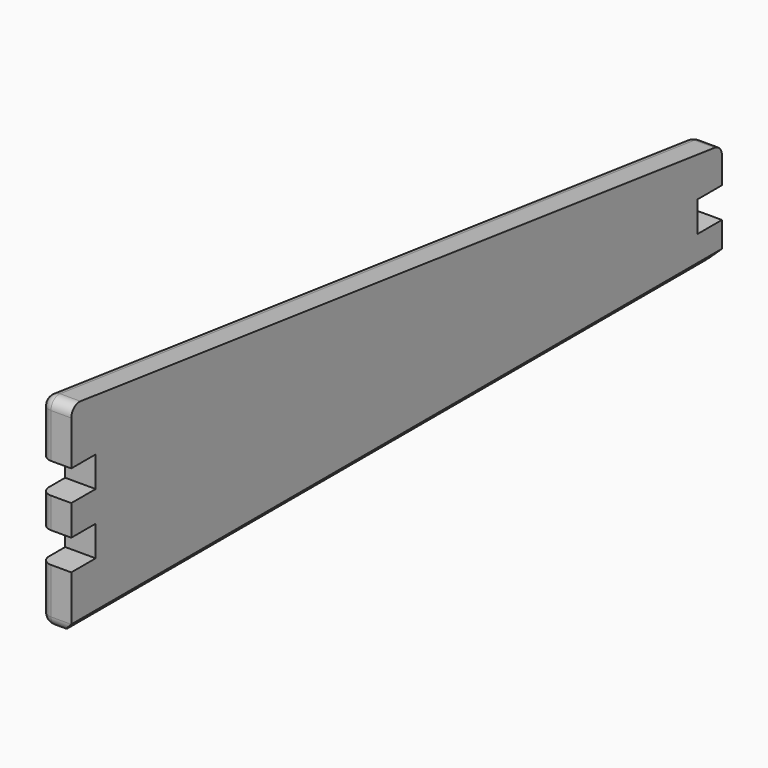
from build123d import *

# Parameters (mm, degrees)
F1_DEPTH     = 15
F2_R         = 5
F3_T1_DEPTH  = 390
F3_T3_DEPTH  = 393.0350652296
F3_T5_DEPTH  = 22.5
F3_T7_DEPTH  = 21.0347777317
F3_T9_DEPTH  = 24.1597777317
F3_T14_DEPTH = 5
F3_T20_DEPTH = 5
F3_T24_ANGLE = 90
F3_T26_ANGLE = 90
F4_T1_DEPTH  = 415.7168298797


# Not quite as in the source:
# - a fillet or chamfer that OpenCascade refuses, or shapes differently, is made with other operations: its cross-section is extruded or revolved along the edge and cut away or added


with BuildPart() as f1:
    # F0 (on Right) → F1 (new body)
    with BuildSketch(Plane.YZ):
        Polygon((-193.8978725672, -35.3695585671), (206.1021274328, -35.3695585671), (206.1021274328, -17.8695585671), (191.1021274328, -17.8695585671), (191.1021274328, -2.8695585671), (206.1021274328, -2.8695585671), (206.1021274328, 14.6304414329), (-193.8978725672, 64.6304414329), (-193.8978725672, 37.1304414329), (-178.8978725672, 37.1304414329), (-178.8978725672, 22.1304414329), (-193.8978725672, 22.1304414329), (-193.8978725672, 7.1304414329), (-178.8978725672, 7.1304414329), (-178.8978725672, -7.8695585671), (-193.8978725672, -7.8695585671), align=None)
    extrude(amount=F1_DEPTH)

    # F2
    f2_edges = [f1.edges().sort_by_distance(p)[0] for p in [
        (0, 206.102127, 5.880441),
        (0, 206.102127, -26.619559),
        (0, -193.897873, 50.880441),
        (0, -193.897873, 14.630441),
        (0, -193.897873, -21.619559),
    ]]
    fillet(f2_edges, radius=F2_R)

    # F3: fillet of radius 5 on 8 edges, made by hand

    # F3_s2 → F3_t1 (cut)
    with BuildSketch(Plane.XZ.offset(-201.1021274328)):
        with BuildLine():
            ThreePointArc((0, -30.3695585671), (1.4644660941, -33.905092473), (5, -35.3695585671))
            Line((5, -35.3695585671), (0, -35.3695585671))
            Line((0, -35.3695585671), (0, -30.3695585671))
        make_face()
    extrude(amount=F3_T1_DEPTH, mode=Mode.SUBTRACT)

    # F3_s4 → F3_t3 (cut)
    with BuildSketch(Plane(origin=(0, 196.7508294304, -24.5938536788), x_dir=(1, 0, 0), z_dir=(0, -0.9922778767, 0.1240347346))):
        with BuildLine():
            ThreePointArc((0, 35.0812860348), (1.4644660941, 38.6168199408), (5, 40.0812860348))
            Line((5, 40.0812860348), (0, 40.0812860348))
            Line((0, 40.0812860348), (0, 35.0812860348))
        make_face()
    extrude(amount=F3_T3_DEPTH, mode=Mode.SUBTRACT)

    # F3_s6 → F3_t5 (cut)
    with BuildSketch(Plane.YZ.offset(5)):
        with BuildLine():
            ThreePointArc((-193.8978725672, -30.3695585671), (-192.4334064731, -33.905092473), (-188.8978725672, -35.3695585671))
            Line((-188.8978725672, -35.3695585671), (-193.8978725672, -35.3695585671))
            Line((-193.8978725672, -35.3695585671), (-193.8978725672, -30.3695585671))
        make_face()
        with BuildLine():
            ThreePointArc((201.1021274328, -35.3695585671), (204.6376613388, -33.905092473), (206.1021274328, -30.3695585671))
            Line((206.1021274328, -30.3695585671), (206.1021274328, -35.3695585671))
            Line((206.1021274328, -35.3695585671), (201.1021274328, -35.3695585671))
        make_face()
    extrude(amount=F3_T5_DEPTH, mode=Mode.SUBTRACT)

    # F3_s8 → F3_t7 (cut)
    with BuildSketch(Plane.YZ.offset(5)):
        with BuildLine():
            ThreePointArc((206.1021274328, 10.2165303402), (204.8505183119, 13.5255431564), (201.7223011058, 15.1779197238))
            Line((201.7223011058, 15.1779197238), (206.1021274328, 14.6304414329))
            Line((206.1021274328, 14.6304414329), (206.1021274328, 10.2165303402))
        make_face()
    extrude(amount=F3_T7_DEPTH, mode=Mode.SUBTRACT)

    # F3_s10 → F3_t9 (cut)
    with BuildSketch(Plane.YZ.offset(5)):
        with BuildLine():
            ThreePointArc((-188.2776988942, 63.9279197238), (-192.2068853834, 62.7149212193), (-193.8978725672, 58.9665303402))
            Line((-193.8978725672, 58.9665303402), (-193.8978725672, 64.6304414329))
            Line((-193.8978725672, 64.6304414329), (-188.2776988942, 63.9279197238))
        make_face()
    extrude(amount=F3_T9_DEPTH, mode=Mode.SUBTRACT)


with BuildPart() as f3_tool12:
    # F3_s13 → F3_t14 (new body)
    with BuildSketch(Plane.YZ.offset(5)):
        Polygon((-188.8978725672, 58.9665303402), (-188.2776988942, 63.9279197238), (-193.8978725672, 64.6304414329), (-193.8978725672, 58.9665303402), align=None)
    extrude(amount=-F3_T14_DEPTH)

    # F3_s15 → F3_t16 (revolve, cut)
    with BuildSketch(Plane(origin=(5, -188.8978725672, 58.9665303402), x_dir=(0, 0.6618025632, -0.7496781758), z_dir=(0, 0.7496781758, 0.6618025632))):
        with BuildLine():
            ThreePointArc((0, -5), (5, 0), (0, 5))
            Line((0, 5), (0, -5))
        make_face()
    revolve(axis=Axis((5, -188.8978725672, 58.9665303402), (-1, 0, 0)), mode=Mode.SUBTRACT)


with BuildPart() as f1_1:
    add(f1.part)

    # F3_t11: cut F3_tool12
    add(f3_tool12.part, mode=Mode.SUBTRACT)


with BuildPart() as f3_tool18:
    # F3_s19 → F3_t20 (new body)
    with BuildSketch(Plane.YZ.offset(5)):
        Polygon((201.1021274328, 10.2165303402), (206.1021274328, 10.2165303402), (206.1021274328, 14.6304414329), (201.7223011058, 15.1779197238), align=None)
    extrude(amount=-F3_T20_DEPTH)

    # F3_s21 → F3_t22 (revolve, cut)
    with BuildSketch(Plane(origin=(5, 201.1021274328, 10.2165303402), x_dir=(0, -0.7496781758, -0.6618025632), z_dir=(0, 0.6618025632, -0.7496781758))):
        with BuildLine():
            ThreePointArc((0, -5), (5, 0), (0, 5))
            Line((0, 5), (0, -5))
        make_face()
    revolve(axis=Axis((5, 201.1021274328, 10.2165303402), (-1, 0, 0)), mode=Mode.SUBTRACT)


with BuildPart() as f1_2:
    add(f1_1.part)

    # F3_t17: cut F3_tool18
    add(f3_tool18.part, mode=Mode.SUBTRACT)

    # F3_s23 → F3_t24 (revolve, cut)
    with BuildSketch(Plane.YZ.offset(5)):
        with BuildLine():
            ThreePointArc((-188.8978725672, -35.3695585671), (-192.4334064731, -33.905092473), (-193.8978725672, -30.3695585671))
            Line((-193.8978725672, -30.3695585671), (-193.8978725672, -35.3695585671))
            Line((-193.8978725672, -35.3695585671), (-188.8978725672, -35.3695585671))
        make_face()
    revolve(axis=Axis((5, -188.8978725672, -35.3695585671), (0, 0, -1)), revolution_arc=F3_T24_ANGLE, mode=Mode.SUBTRACT)

    # F3_s25 → F3_t26 (revolve, cut)
    with BuildSketch(Plane.YZ.offset(5)):
        with BuildLine():
            ThreePointArc((201.1021274328, -35.3695585671), (204.6376613388, -33.905092473), (206.1021274328, -30.3695585671))
            Line((206.1021274328, -30.3695585671), (206.1021274328, -35.3695585671))
            Line((206.1021274328, -35.3695585671), (201.1021274328, -35.3695585671))
        make_face()
    revolve(axis=Axis((5, 201.1021274328, -35.3695585671), (0, 0, 1)), revolution_arc=F3_T26_ANGLE, mode=Mode.SUBTRACT)

    # F4: chamfer of 5 on 1 edges, made by hand

    # F4_s2 → F4_t1 (cut)
    with BuildSketch(Plane.XZ.offset(-213.9605423726)):
        Polygon((15, -30.3695585671), (10, -35.3695585671), (15, -35.3695585671), align=None)
    extrude(amount=F4_T1_DEPTH, mode=Mode.SUBTRACT)


solid = f1_2.part
